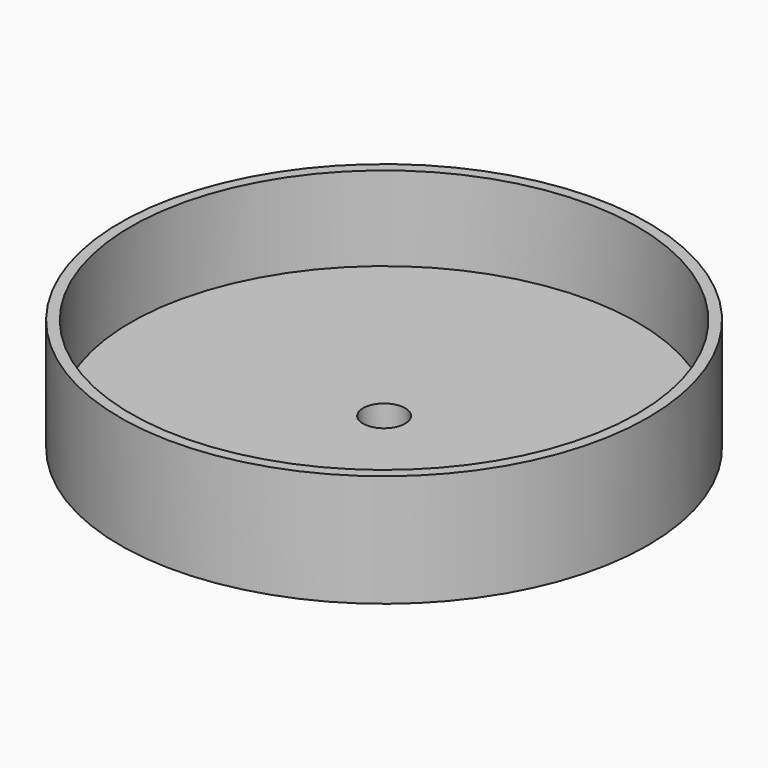
from build123d import *

# Parameters (mm, degrees)
F0_R     = 59.69
F1_DEPTH = 6.35
F2_R     = 59.69
F2_R_2   = 57.277
F3_DEPTH = 19.05
F4_R     = 4.7625
F5_DEPTH = 25.4


# Not quite as in the source:
# - a feature names something its author has since deleted; it is built from what else it names


with BuildPart() as f1:
    # F0 (on Top) → F1 (new body)
    with BuildSketch(Plane.XY):
        Circle(F0_R)
    extrude(amount=F1_DEPTH)

    # F2 (on face) → F3 (join)
    with BuildSketch(Plane.XY.offset(6.35)):
        Circle(F2_R)
        Circle(F2_R_2, mode=Mode.SUBTRACT)
    extrude(amount=F3_DEPTH)

    # F4 (on face) → F5 (cut)
    with BuildSketch(Plane.XY.offset(6.35)):
        Circle(F4_R)
    extrude(amount=-F5_DEPTH, mode=Mode.SUBTRACT)


solid = f1.part
